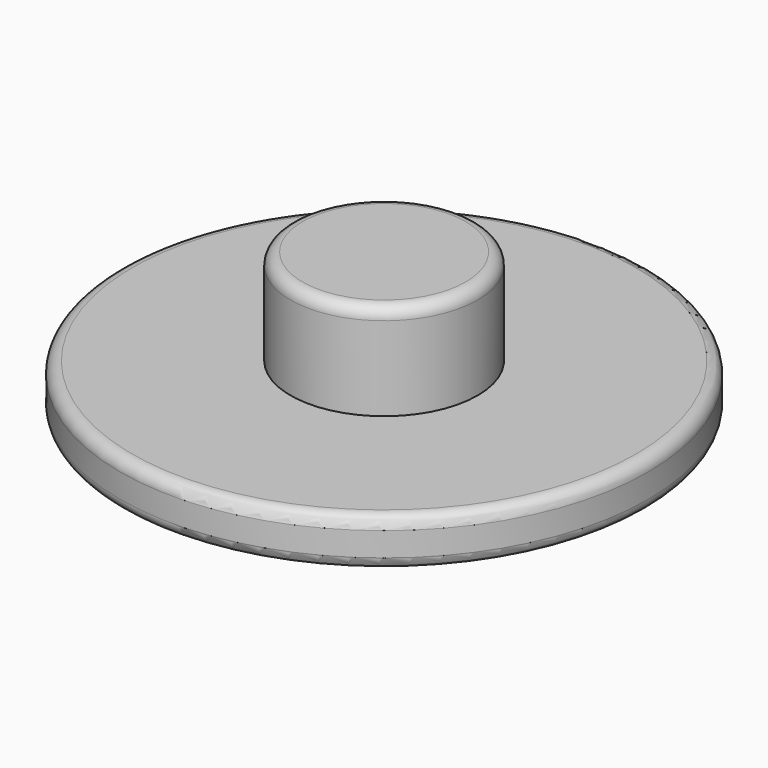
from build123d import *

# Parameters (mm, degrees)
F0_R     = 11
F1_DEPTH = 2
F2_R     = 3.9
F3_DEPTH = 6
F4_R     = 0.5


# Not quite as in the source:
# - a feature names something its author has since deleted; it is built from what else it names


with BuildPart() as f1:
    # F0 (on Top) → F1 (new body)
    with BuildSketch(Plane.XY):
        Circle(F0_R)
    extrude(amount=F1_DEPTH)

    # F2 (on Top) → F3 (join)
    with BuildSketch(Plane.XY):
        Circle(F2_R)
    extrude(amount=F3_DEPTH)

    # F4
    f4_edges = [f1.edges().sort_by_distance(p)[0] for p in [
        (-11, 0, 2),
        (-11, 0, 0),
        (-3.9, 0, 6),
    ]]
    fillet(f4_edges, radius=F4_R)


solid = f1.part
